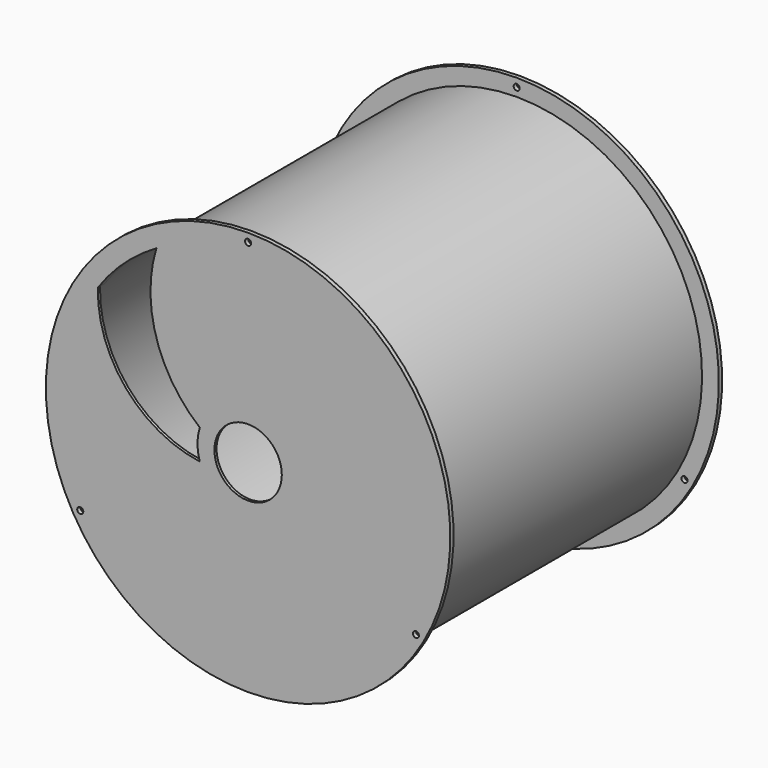
from build123d import *

# Parameters (mm, degrees)
F2_R            = 100
F3_DEPTH        = 25
F4_R            = 9
F5_DEPTH        = 1008.001
F5_COPIES_COUNT = 3
F7_DEPTH        = 25


# Not quite as in the source:
# - a pattern or mirror of a feature is missing from the dataset's text; its kind, count and spacing are read off the source's solid


with BuildPart() as f1:
    # F0 (on Right) → F1 (revolve)
    with BuildSketch(Plane.YZ):
        Polygon((12, 600), (0, 600), (0, 0), (8, 0), (8, 544), (1008, 544), (1008, 600), (996, 600), (996, 550), (12, 550), align=None)
    revolve(axis=Axis((0, 4, 0), (0, -1, 0)))

    # F2 (on face) → F3 (cut)
    with BuildSketch(Plane.XZ):
        Circle(F2_R)
    extrude(amount=-F3_DEPTH, mode=Mode.SUBTRACT)

    # F4 (on face) → F5 (cut, through all)
    with BuildSketch(Plane.XZ):
        with Locations((0, 575)):
            Circle(F4_R)
    f5 = extrude(amount=-F5_DEPTH, mode=Mode.SUBTRACT)

    # F5_copies: F5 ×3 about axis
    f5_copies_axis = Axis((0, 0, 0), (0, 1, 0))
    for i in range(1, F5_COPIES_COUNT):
        add(f5.rotate(f5_copies_axis, i * 360 / F5_COPIES_COUNT), mode=Mode.SUBTRACT)

    # F6 (on face) → F7 (cut)
    with BuildSketch(Plane.XZ):
        with BuildLine():
            ThreePointArc((-143.2870199028, 44.3714990436), (-272.593694434, 238.1547264126), (-272, 471.1178196587))
            ThreePointArc((-272, 471.1178196587), (-367.5210729429, 401.0788712247), (-445.6187120932, 312.025581375))
            ThreePointArc((-445.6187120932, 312.025581375), (-362.6540145598, 75.9719974886), (-143.2870199028, -44.3714990436))
            ThreePointArc((-143.2870199028, -44.3714990436), (-150, 0), (-143.2870199028, 44.3714990436))
        make_face()
    extrude(amount=-F7_DEPTH, mode=Mode.SUBTRACT)


solid = f1.part
